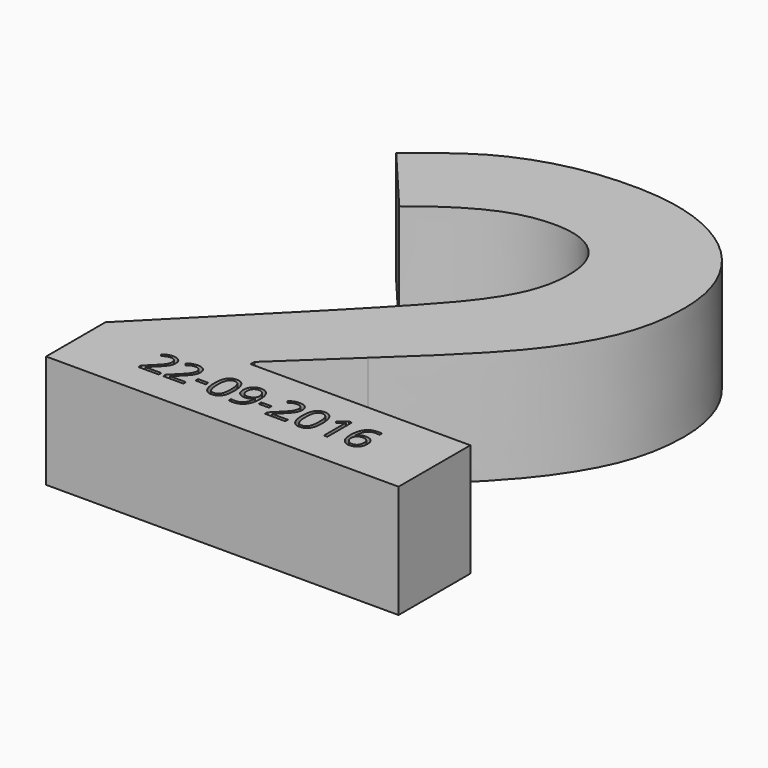
from build123d import *

# Parameters (mm, degrees)
F0_TEXT_SIZE = 250
F1_DEPTH     = 40
F2_TEXT_SIZE = 15.2867763413
F3_DEPTH     = 3


# Not quite as in the source:
# - Text() gives the source's letters only with a copy of the font that has no kerning and outlines rounded to 1/6400 em; it was checked with that copy


with BuildPart() as f1:
    # F0 (on Top) → F1 (new body)
    with BuildSketch(Plane.XY):
        with Locations((-99.3761267545, -85.9230706586)):
            Text('2', F0_TEXT_SIZE, font='Open Sans', font_style=FontStyle.BOLD, text_align=(TextAlign.LEFT, TextAlign.BOTTOM))
    extrude(amount=F1_DEPTH)

    # F2 (on face) → F3 (cut)
    with BuildSketch(Plane.XY.offset(40)):
        with Locations((-66.263495464, -74.8913709054)):
            Text('22-09-2016', F2_TEXT_SIZE, font='Open Sans', text_align=(TextAlign.LEFT, TextAlign.BOTTOM))
    extrude(amount=-F3_DEPTH, mode=Mode.SUBTRACT)


solid = f1.part
